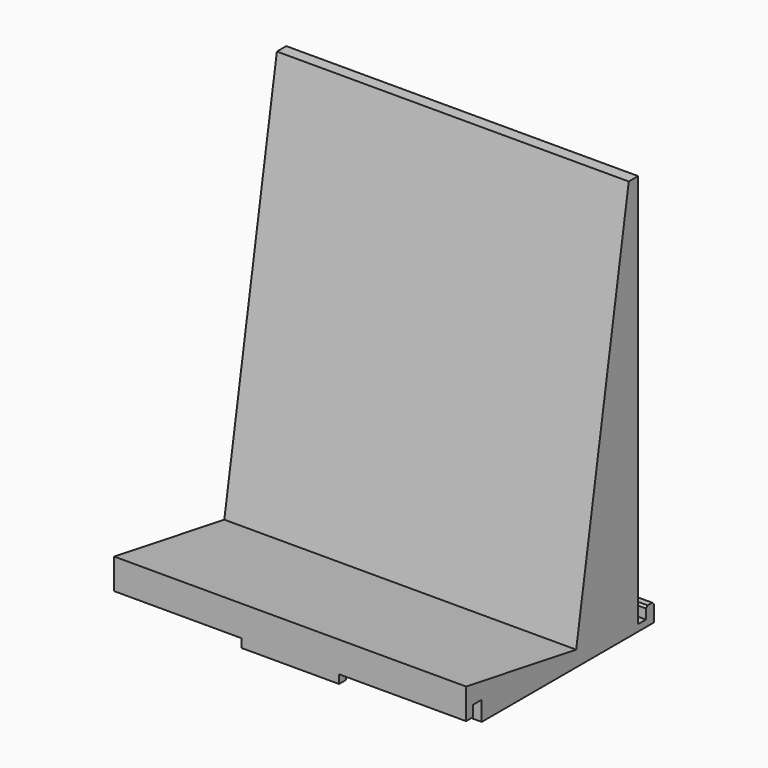
from build123d import *

# Parameters (mm, degrees)
F0_W      = 90
F0_H      = 60
F1_DEPTH  = 4
F3_DEPTH  = 90
F4_W      = 2.2
F4_H      = 2.2
F4_W_2    = 2.5
F4_H_2    = 2.3
F5_DEPTH  = 90
F4_H_3    = 0.7
F6_DEPTH  = 90
F7_W      = 25
F7_H      = 2.2
F8_DEPTH  = 2.2
F9_W      = 26
F9_H      = 2.5
F10_DEPTH = 1.7
F11_SIZE  = 0.5


with BuildPart() as f1:
    # F0 (on Top) → F1 (new body)
    with BuildSketch(Plane.XY):
        Rectangle(F0_W, F0_H)
    extrude(amount=F1_DEPTH)

    # F2 (on face) → F3 (join, through all)
    with BuildSketch(Plane.YZ.offset(45)):
        Polygon((22, 102.5777145975), (5.1942216862, 4), (25, 4), (25, 102.5777145975), align=None)
        Polygon((-30, 10), (-30, 4), (5.1942216862, 4), align=None)
    extrude(amount=-F3_DEPTH)

    # F4 (on face) → F5 (cut, through all)
    with BuildSketch(Plane.YZ.offset(45)):
        with Locations((-28.9, 1.1)):
            Rectangle(F4_W, F4_H)
        Polygon((-27.8, 2.2), (-27.8, 0), (-25, 0), (-25, 5), (-27.8, 5), align=None)
        with Locations((26.25, 2.85)):
            Rectangle(F4_W_2, F4_H_2)
    extrude(amount=-F5_DEPTH, mode=Mode.SUBTRACT)

    # F4 (on face) → F6 (join, through all)
    with BuildSketch(Plane.YZ.offset(45)):
        with Locations((28.75, 4.35)):
            Rectangle(F4_W_2, F4_H_3)
    extrude(amount=-F6_DEPTH)

    # F7 (on face) → F8 (join, through all)
    with BuildSketch(Plane(origin=(0, 0, 2.2), x_dir=(1, 0, 0), z_dir=(0, 0, -1))):
        with Locations((0, 28.9)):
            Rectangle(F7_W, F7_H)
    extrude(amount=F8_DEPTH)

    # F9 (on face) → F10 (cut, through all)
    with BuildSketch(Plane.XY.offset(1.7)):
        with Locations((0, 26.25)):
            Rectangle(F9_W, F9_H)
    extrude(amount=-F10_DEPTH, mode=Mode.SUBTRACT)

    # F11
    f11_edges = [f1.edges().sort_by_distance(p)[0] for p in [
        (0, 30, 4.7),
        (0, 27.5, 4.7),
        (-13, 26.25, 1.7),
        (13, 26.25, 1.7),
    ]]
    chamfer(f11_edges, length=F11_SIZE)


solid = f1.part
